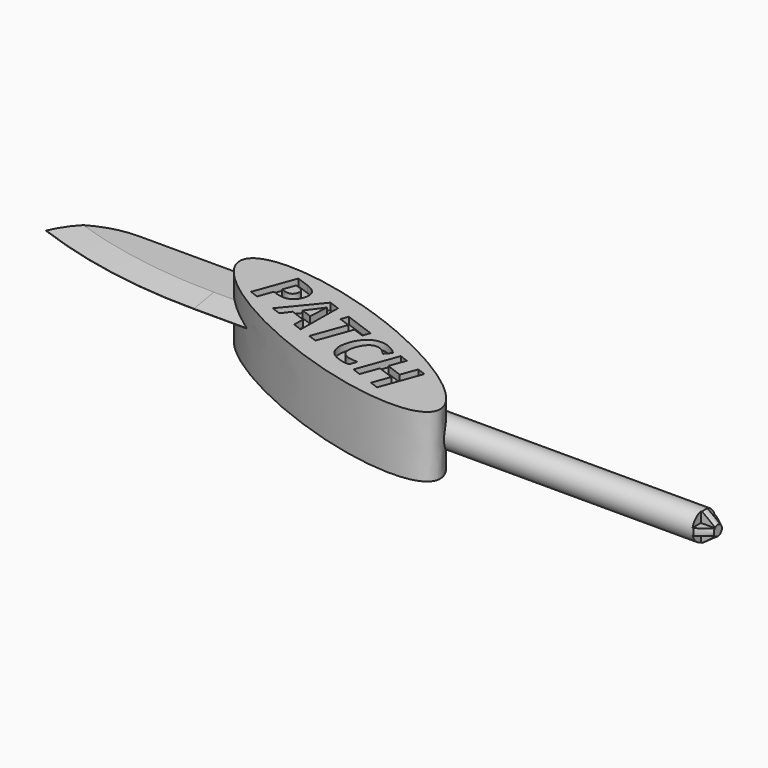
from build123d import *

# Parameters (mm, degrees)
F1_DEPTH      = 13.716
F2_R          = 3.175
F3_DEPTH      = 64.262
F4_DEPTH      = 25.4
F6_DEPTH      = 3.175
F7_SIZE2      = 2.032
F7_SIZE       = 2.9019967497
F8_W          = 13.97
F8_H          = 2.032
F9_DEPTH      = 71.374
F11_DEPTH     = 10.668
F12_SIZE2     = 5.588
F12_SIZE      = 0.9853151682
F13_TEXT_SIZE = 13.5770534052
F14_DEPTH     = 1.524
F15_DEPTH     = 25.4


# Not quite as in the source:
# - Text() gives the source's letters only with a copy of the font that has no kerning and outlines rounded to 1/6400 em; it was checked with that copy


with BuildPart() as f1:
    # F0 (on Top) → F1 (new body)
    with BuildSketch(Plane.XY):
        with BuildLine():
            add(Edge.make_bspline(
                [(-3.7550868284, 11.1494023457), (-28.3637118551, 18.8621042303), (-31.021842733, 11.9775449857)],
                knots=[4.9404677153, 4.9404677153, 4.9404677153, 6.2831853072, 6.2831853072, 6.2831853072], degree=2, weights=[1, 0.7829771493, 1]))
            add(Edge.make_bspline(
                [(-31.021842733, 11.9775449857), (-39.7556801434, -10.6430947969), (20.8465143723, -14.7016081621), (81.4487088881, -18.7601215274), (0, 9.9000201642)],
                knots=[0, 0, 0, 2.4099133424, 2.4099133424, 4.8198266848, 4.8198266848, 4.8198266848], degree=2, weights=[1, 0.3577335108, 1, 0.3577335108, 1]))
            add(Edge.make_bspline(
                [(0, 9.9000201642), (-1.8843915827, 10.5630991804), (-3.7550868284, 11.1494023457)],
                knots=[4.8198266848, 4.8198266848, 4.8198266848, 4.9404677153, 4.9404677153, 4.9404677153], degree=2, weights=[1, 0.9981812693, 1]))
        make_face()
    extrude(amount=F1_DEPTH)

    # F2 (on Right) → F3 (join)
    with BuildSketch(Plane.YZ):
        with Locations((-6.3480981626, 6.9469762966)):
            Circle(F2_R)
    extrude(amount=F3_DEPTH)

    # F4 (add): a face of the model
    f4_faces = [f1.faces().sort_by_distance(p)[0] for p in [
        (64.262, -6.3480981626, 6.9469762966),
    ]]
    extrude(f4_faces, amount=F4_DEPTH)

    # F5 (on face) → F6 (cut)
    with BuildSketch(Plane.YZ.offset(89.662)):
        with BuildLine():
            ThreePointArc((-3.2658942433, 7.7089762966), (-4.1030341323, 9.1920403269), (-5.5860981626, 10.0291802159))
            Line((-5.5860981626, 10.0291802159), (-5.5860981626, 7.7089762966))
            Line((-5.5860981626, 7.7089762966), (-3.2658942433, 7.7089762966))
        make_face()
        with BuildLine():
            Line((-7.1100981626, 7.7089762966), (-7.1100981626, 10.0291802159))
            ThreePointArc((-7.1100981626, 10.0291802159), (-8.5931621928, 9.1920403269), (-9.4303020818, 7.7089762966))
            Line((-9.4303020818, 7.7089762966), (-7.1100981626, 7.7089762966))
        make_face()
        with BuildLine():
            Line((-7.1100981626, 6.1849762966), (-9.4303020818, 6.1849762966))
            ThreePointArc((-9.4303020818, 6.1849762966), (-8.5931621928, 4.7019122663), (-7.1100981626, 3.8647723773))
            Line((-7.1100981626, 3.8647723773), (-7.1100981626, 6.1849762966))
        make_face()
        with BuildLine():
            ThreePointArc((-5.5860981626, 3.8647723773), (-4.1030341323, 4.7019122663), (-3.2658942433, 6.1849762966))
            Line((-3.2658942433, 6.1849762966), (-5.5860981626, 6.1849762966))
            Line((-5.5860981626, 6.1849762966), (-5.5860981626, 3.8647723773))
        make_face()
    extrude(amount=-F6_DEPTH, mode=Mode.SUBTRACT)

    # F7
    f7_edges = [f1.edges().sort_by_distance(p)[0] for p in [
        (89.662, -9.523098, 6.946976),
        (89.662, -6.348098, 3.771976),
        (89.662, -3.196383, 7.330791),
        (89.662, -6.348098, 10.121976),
    ]]
    f7_side = f1.faces().sort_by_distance((57.521666, -9.523098, 6.946976))[0]
    chamfer(f7_edges, length=F7_SIZE, length2=F7_SIZE2, reference=f7_side)

    # F8 (on Right) → F9 (join)
    with BuildSketch(Plane.YZ):
        with Locations((6.985, 8.2377603743)):
            Rectangle(F8_W, F8_H)
    extrude(amount=-F9_DEPTH)

    # F10 (on face) → F11 (cut)
    with BuildSketch(Plane(origin=(0, 0, 7.2217603743), x_dir=(1, 0, 0), z_dir=(0, 0, -1))):
        with BuildLine():
            ThreePointArc((-56.1839674742, -13.97), (-64.5435026457, -12.1400722389), (-71.374, -6.985))
            Line((-71.374, -6.985), (-71.374, -13.97))
            Line((-71.374, -13.97), (-56.1839674742, -13.97))
        make_face()
        with BuildLine():
            Line((-71.374, 0), (-71.374, -6.985))
            ThreePointArc((-71.374, -6.985), (-52.3539747529, -1.7602691464), (-32.7080941306, 0))
            Line((-32.7080941306, 0), (-71.374, 0))
        make_face()
    extrude(amount=-F11_DEPTH, mode=Mode.SUBTRACT)

    # F12
    f12_edges = [f1.edges().sort_by_distance(p)[0] for p in [
        (-52.353975, 1.760269, 7.22176),
        (-52.353975, 1.760269, 9.25376),
    ]]
    f12_side = f1.faces().sort_by_distance((-52.353975, 1.760269, 8.23776))[0]
    chamfer(f12_edges, length=F12_SIZE, length2=F12_SIZE2, reference=f12_side)

    # F13 (on face) → F14 (cut)
    with BuildSketch(Plane.XY.offset(13.716)):
        with Locations(Location((-23.5227475351, 3.4954527196), (0, 0, -20))):
            Text('PATCH', F13_TEXT_SIZE, font='Open Sans', font_style=FontStyle.BOLD, text_align=(TextAlign.LEFT, TextAlign.BOTTOM))
    extrude(amount=-F14_DEPTH, mode=Mode.SUBTRACT)

    # F15 (cut): a face of the model
    f15_faces = [f1.faces().sort_by_distance(p)[0] for p in [
        (-4.7111000109, 12.6753032572, 9.2537603743),
    ]]
    extrude(f15_faces, amount=-F15_DEPTH, mode=Mode.SUBTRACT)


solid = f1.part
